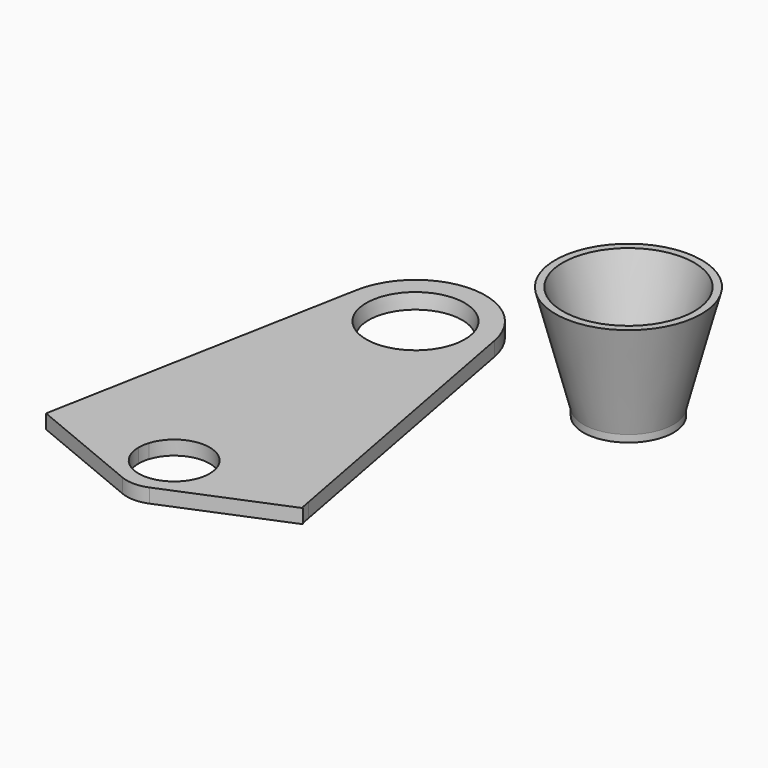
from build123d import *

# Parameters (mm, degrees)
F0_R     = 13
F1_DEPTH = 4


# Not quite as in the source:
# - a fillet or chamfer that OpenCascade refuses, or shapes differently, is made with other operations: its cross-section is extruded or revolved along the edge and cut away or added


with BuildPart() as f1:
    # F0 (on Top) → F1 (new body)
    with BuildSketch(Plane.XY):
        with BuildLine():
            Line((-36.0218728627, -85), (-10, -85))
            ThreePointArc((-10, -85), (-9.8841772582, -83.4824230072), (-9.5393920142, -82))
            Line((-9.5393920142, -82), (-35.4579826076, -82))
            Line((-35.4579826076, -82), (-36.0218728627, -85))
        make_face()
        with BuildLine():
            Line((10, -85), (36.0218728627, -85))
            Line((36.0218728627, -85), (35.4579826076, -82))
            Line((35.4579826076, -82), (9.5393920142, -82))
            ThreePointArc((9.5393920142, -82), (9.8841772582, -83.4824230072), (10, -85))
        make_face()
        with BuildLine():
            Line((9.5393920142, -82), (35.4579826076, -82))
            Line((35.4579826076, -82), (19.3609549854, 3.6391512822))
            ThreePointArc((19.3609549854, 3.6391512822), (0, 19.7), (-19.3609549854, 3.6391512822))
            Line((-19.3609549854, 3.6391512822), (-35.4579826076, -82))
            Line((-35.4579826076, -82), (-9.5393920142, -82))
            ThreePointArc((-9.5393920142, -82), (0, -75), (9.5393920142, -82))
        make_face()
        Circle(F0_R, mode=Mode.SUBTRACT)
        with BuildLine():
            Line((3.8250876827, -98.4205655408), (36.3271264003, -85))
            Line((36.3271264003, -85), (36.0218728627, -85))
            Line((36.0218728627, -85), (10, -85))
            ThreePointArc((10, -85), (0, -95), (-10, -85))
            Line((-10, -85), (-36.0218728627, -85))
            Line((-36.0218728627, -85), (-36.0322895223, -85.0554185474))
            Line((-36.0322895223, -85.0554185474), (-3.822600818, -98.4145562205))
            ThreePointArc((-3.822600818, -98.4145562205), (0.0006462735, -99.1775278473), (3.8250876827, -98.4205655408))
        make_face()
    extrude(amount=F1_DEPTH)

    # F4: chamfer of 5 x 0.8816349035 on 1 edges, made by hand

    # F4_s1 → F4_t2 (revolve, cut)
    with BuildSketch(Plane.XZ):
        Polygon((13, -1), (13.8816349035, 4), (13, 4), align=None)
    revolve(axis=Axis((0, 0, 4), (0, 0, 1)), mode=Mode.SUBTRACT)


with BuildPart() as f3:
    # F2 (on Front) → F3 (revolve)
    with BuildSketch(Plane.XZ):
        Polygon((60, 2), (60, 0), (72.7, 0), (72.7, 2), (80.5971898989, 32), (78.5290553575, 32), (70.6318654586, 2), align=None)
    revolve(axis=Axis((60, 0, 12.6420042982), (0, 0, 1)))


solid = Compound([f1.part, f3.part])
